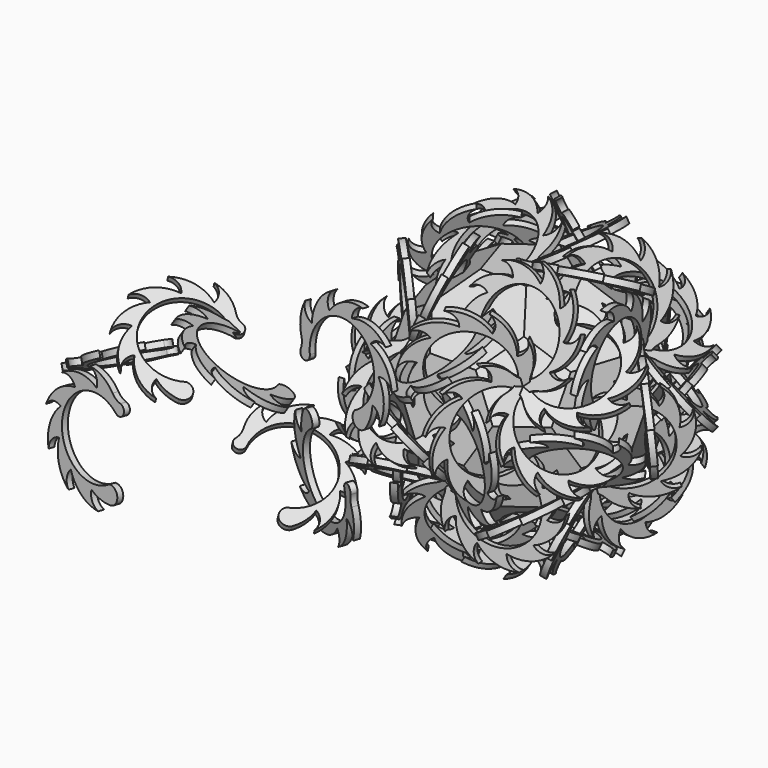
from build123d import *

# Parameters (mm, degrees)
F2_DEPTH  = 1
F3_DEPTH  = 1
F4_ANGLE  = -37.377368
F6_COUNT  = 5
F6_ANGLE  = 288
F9_DEPTH  = 2
F10_R     = 5.4550197089
F12_ANGLE = 65
F13_COUNT = 5
F13_ANGLE = 288
F15_COUNT = 3
F15_ANGLE = 240
F16_COUNT = 5
F16_ANGLE = 288
F17_COUNT = 2
F17_ANGLE = 120
F18_COUNT = 3
F18_ANGLE = 240
F22_COUNT = 3
F22_ANGLE = 144
F26_COUNT = 3
F26_ANGLE = 144
F29_COUNT = 2
F29_ANGLE = 120
F32_COUNT = 3
F32_ANGLE = 144
F36_COUNT = 3
F36_ANGLE = 240
F40_COUNT = 3
F40_ANGLE = 144
F44_COUNT = 3
F44_ANGLE = 144
F48_COUNT = 2
F48_ANGLE = 120
F52_COUNT = 2
F52_ANGLE = 120
F56_COUNT = 2
F56_ANGLE = 120
F60_COUNT = 2
F60_ANGLE = 120


with BuildPart() as f2:
    # F0 (on Top) → F2 (new body)
    with BuildSketch(Plane.XY):
        Polygon((0, -10.3228644035), (7.5, -10.3228644035), (12.1352549156, 3.9429833409), (0, 12.7597621253), align=None)
        Polygon((-7.5, -10.3228644035), (0, -10.3228644035), (0, 12.7597621253), (-12.1352549156, 3.9429833409), align=None)
    extrude(amount=-F2_DEPTH)


with BuildPart() as f3:
    # F1 (on Top) → F3 (new body)
    with BuildSketch(Plane.XY):
        Polygon((32.2091731064, -18.3513614234), (36.844428022, -4.085513679), (26.8074689266, 7.0616587032), (12.1352549156, 3.9429833409), (7.5, -10.3228644035), (17.5369590954, -21.4700367857), align=None)
    extrude(amount=-F3_DEPTH)


with BuildPart() as f3_1:
    # F4: moved
    add(f3.part.rotate(Axis((9.8176274578, -3.1899405313, 0), (-0.3090169944, -0.9510565163, 0)), F4_ANGLE))


with BuildPart() as f6_1:
    # F6: instance of F3
    add(f3_1.part.rotate(Axis((0, 0, 3.8664315362), (0, 0, 1)), 1 * F6_ANGLE / (F6_COUNT - 1)))


with BuildPart() as f6_2:
    # F6: instance of F3
    add(f3_1.part.rotate(Axis((0, 0, 3.8664315362), (0, 0, 1)), 2 * F6_ANGLE / (F6_COUNT - 1)))


with BuildPart() as f6_3:
    # F6: instance of F3
    add(f3_1.part.rotate(Axis((0, 0, 3.8664315362), (0, 0, 1)), 3 * F6_ANGLE / (F6_COUNT - 1)))


with BuildPart() as f6_4:
    # F6: instance of F3
    add(f3_1.part.rotate(Axis((0, 0, 3.8664315362), (0, 0, 1)), 4 * F6_ANGLE / (F6_COUNT - 1)))


with BuildPart() as f9:
    # F8 (on Right) → F9 (new body)
    with BuildSketch(Plane.YZ):
        with BuildLine():
            ThreePointArc((-20.0381562793, -7.4218225341), (-18.0432138806, 14.7456768661), (-1.371596125, 0))
            ThreePointArc((-1.371596125, 0), (1.2710572909, -2.1110060804), (1.0658705895, 1.265065922))
            ThreePointArc((1.0658705895, 1.265065922), (3.462744203, 7.3677169674), (2.5001799222, 13.8531485572))
            ThreePointArc((2.5001799222, 13.8531485572), (1.8396441745, 10.7438611605), (-0.8004298525, 8.9735547684))
            ThreePointArc((-0.8004298525, 8.9735547684), (-2.1304901639, 15.9377846017), (-6.983453041, 21.1067602176))
            ThreePointArc((-6.983453041, 21.1067602176), (-5.7243130519, 18.2607184854), (-6.7542303289, 15.3239417734))
            ThreePointArc((-6.7542303289, 15.3239417734), (-11.923743314, 20.1763322255), (-18.8881203911, 21.5056213332))
            ThreePointArc((-18.8881203911, 21.5056213332), (-16.196593384, 19.9432291213), (-15.3036199233, 16.9619566661))
            ThreePointArc((-15.3036199233, 16.9619566661), (-22.3380073271, 17.8490595111), (-28.7536432712, 14.8309188523))
            ThreePointArc((-28.7536432712, 14.8309188523), (-25.6578010812, 15.1489568819), (-23.1830223937, 13.2619334316))
            ThreePointArc((-23.1830223937, 13.2619334316), (-29.3953873179, 9.8449055341), (-32.8117272579, 3.6321622578))
            ThreePointArc((-32.8117272579, 3.6321622578), (-30.4940763777, 5.7091508113), (-27.3827738075, 5.6371551864))
            ThreePointArc((-27.3827738075, 5.6371551864), (-30.4002040016, -0.7788149372), (-29.5123221974, -7.813104063))
            ThreePointArc((-29.5123221974, -7.813104063), (-28.8581264893, -4.7705040188), (-26.2987118688, -2.9999719366))
            ThreePointArc((-26.2987118688, -2.9999719366), (-26.0274642787, -7.0575500385), (-24.4889350399, -10.821914937))
            ThreePointArc((-24.4889350399, -10.821914937), (-20.5634994581, -11.3472581158), (-20.0381562793, -7.4218225341))
        make_face()
    extrude(amount=-F9_DEPTH)

    # F10
    f10_edges = [f9.edges().sort_by_distance(p)[0] for p in [
        (-1, 1.065871, 1.265066),
    ]]
    fillet(f10_edges, radius=F10_R)


with BuildPart() as f9_1:
    # F12: moved
    add(f9.part.rotate(Axis((0, -10.3228644132, -3.9429833282), (0, -0.9341723595, -0.3568220885)), F12_ANGLE))


with BuildPart() as f13_1:
    # F13: instance of F9
    add(f9_1.part.rotate(Axis((0, 0, 14.2103461549), (0, 0, 1)), 1 * F13_ANGLE / (F13_COUNT - 1)))


with BuildPart() as f13_2:
    # F13: instance of F9
    add(f9_1.part.rotate(Axis((0, 0, 14.2103461549), (0, 0, 1)), 2 * F13_ANGLE / (F13_COUNT - 1)))


with BuildPart() as f13_3:
    # F13: instance of F9
    add(f9_1.part.rotate(Axis((0, 0, 14.2103461549), (0, 0, 1)), 3 * F13_ANGLE / (F13_COUNT - 1)))


with BuildPart() as f13_4:
    # F13: instance of F9
    add(f9_1.part.rotate(Axis((0, 0, 14.2103461549), (0, 0, 1)), 4 * F13_ANGLE / (F13_COUNT - 1)))


with BuildPart() as f15_1:
    # F15: instance of F9
    add(f9_1.part.rotate(Axis((0, -25.3455492518, -1.7338218178), (0, -0.6070619963, 0.7946544738)), 1 * F15_ANGLE / (F15_COUNT - 1)))


with BuildPart() as f15_2:
    # F15: instance of F9
    add(f9_1.part.rotate(Axis((0, -25.3455492518, -1.7338218178), (0, -0.6070619963, 0.7946544738)), 2 * F15_ANGLE / (F15_COUNT - 1)))


with BuildPart() as f16_1:
    # F16: instance of F15_2
    add(f15_2.part.rotate(Axis((0, 0, 14.2103461549), (0, 0, 1)), 1 * F16_ANGLE / (F16_COUNT - 1)))


with BuildPart() as f16_2:
    # F16: instance of F15_2
    add(f15_2.part.rotate(Axis((0, 0, 14.2103461549), (0, 0, 1)), 2 * F16_ANGLE / (F16_COUNT - 1)))


with BuildPart() as f16_3:
    # F16: instance of F15_2
    add(f15_2.part.rotate(Axis((0, 0, 14.2103461549), (0, 0, 1)), 3 * F16_ANGLE / (F16_COUNT - 1)))


with BuildPart() as f16_4:
    # F16: instance of F15_2
    add(f15_2.part.rotate(Axis((0, 0, 14.2103461549), (0, 0, 1)), 4 * F16_ANGLE / (F16_COUNT - 1)))


with BuildPart() as f16_5:
    # F16: instance of F15_1
    add(f15_1.part.rotate(Axis((0, 0, 14.2103461549), (0, 0, 1)), 1 * F16_ANGLE / (F16_COUNT - 1)))


with BuildPart() as f16_6:
    # F16: instance of F15_1
    add(f15_1.part.rotate(Axis((0, 0, 14.2103461549), (0, 0, 1)), 2 * F16_ANGLE / (F16_COUNT - 1)))


with BuildPart() as f16_7:
    # F16: instance of F15_1
    add(f15_1.part.rotate(Axis((0, 0, 14.2103461549), (0, 0, 1)), 3 * F16_ANGLE / (F16_COUNT - 1)))


with BuildPart() as f16_8:
    # F16: instance of F15_1
    add(f15_1.part.rotate(Axis((0, 0, 14.2103461549), (0, 0, 1)), 4 * F16_ANGLE / (F16_COUNT - 1)))


with BuildPart() as f17_1:
    # F17: instance of F3
    add(f3_1.part.rotate(Axis((0, -25.3455492518, -1.7338218178), (0, 0.6070619963, -0.7946544738)), 1 * F17_ANGLE / (F17_COUNT - 1)))


with BuildPart() as f17_2:
    # F17: instance of F16_5
    add(f16_5.part.rotate(Axis((0, -25.3455492518, -1.7338218178), (0, 0.6070619963, -0.7946544738)), 1 * F17_ANGLE / (F17_COUNT - 1)))


with BuildPart() as f17_3:
    # F17: instance of F13_1
    add(f13_1.part.rotate(Axis((0, -25.3455492518, -1.7338218178), (0, 0.6070619963, -0.7946544738)), 1 * F17_ANGLE / (F17_COUNT - 1)))


with BuildPart() as f17_4:
    # F17: instance of F16_1
    add(f16_1.part.rotate(Axis((0, -25.3455492518, -1.7338218178), (0, 0.6070619963, -0.7946544738)), 1 * F17_ANGLE / (F17_COUNT - 1)))


with BuildPart() as f18_1:
    # F18: instance of F2
    add(f2.part.rotate(Axis((0, -25.3455492518, -1.7338218178), (0, -0.6070619963, 0.7946544738)), 1 * F18_ANGLE / (F18_COUNT - 1)))


with BuildPart() as f18_2:
    # F18: instance of F2
    add(f2.part.rotate(Axis((0, -25.3455492518, -1.7338218178), (0, -0.6070619963, 0.7946544738)), 2 * F18_ANGLE / (F18_COUNT - 1)))


with BuildPart() as f18_3:
    # F18: instance of F13_2
    add(f13_2.part.rotate(Axis((0, -25.3455492518, -1.7338218178), (0, -0.6070619963, 0.7946544738)), 1 * F18_ANGLE / (F18_COUNT - 1)))


with BuildPart() as f18_4:
    # F18: instance of F13_2
    add(f13_2.part.rotate(Axis((0, -25.3455492518, -1.7338218178), (0, -0.6070619963, 0.7946544738)), 2 * F18_ANGLE / (F18_COUNT - 1)))


with BuildPart() as f18_5:
    # F18: instance of F13_3
    add(f13_3.part.rotate(Axis((0, -25.3455492518, -1.7338218178), (0, -0.6070619963, 0.7946544738)), 1 * F18_ANGLE / (F18_COUNT - 1)))


with BuildPart() as f18_6:
    # F18: instance of F13_3
    add(f13_3.part.rotate(Axis((0, -25.3455492518, -1.7338218178), (0, -0.6070619963, 0.7946544738)), 2 * F18_ANGLE / (F18_COUNT - 1)))


with BuildPart() as f22_1:
    # F22: instance of F17_1
    add(f17_1.part.rotate(Axis((-18.9711930891, -26.1116072266, -18.7737157723), (0.5257311104, 0.7236067968, -0.4472135991)), 1 * F22_ANGLE / (F22_COUNT - 1)))


with BuildPart() as f22_2:
    # F22: instance of F17_1
    add(f17_1.part.rotate(Axis((-18.9711930891, -26.1116072266, -18.7737157723), (0.5257311104, 0.7236067968, -0.4472135991)), 2 * F22_ANGLE / (F22_COUNT - 1)))


with BuildPart() as f22_3:
    # F22: instance of F17_3
    add(f17_3.part.rotate(Axis((-18.9711930891, -26.1116072266, -18.7737157723), (0.5257311104, 0.7236067968, -0.4472135991)), 1 * F22_ANGLE / (F22_COUNT - 1)))


with BuildPart() as f22_4:
    # F22: instance of F17_3
    add(f17_3.part.rotate(Axis((-18.9711930891, -26.1116072266, -18.7737157723), (0.5257311104, 0.7236067968, -0.4472135991)), 2 * F22_ANGLE / (F22_COUNT - 1)))


with BuildPart() as f22_5:
    # F22: instance of F17_4
    add(f17_4.part.rotate(Axis((-18.9711930891, -26.1116072266, -18.7737157723), (0.5257311104, 0.7236067968, -0.4472135991)), 1 * F22_ANGLE / (F22_COUNT - 1)))


with BuildPart() as f22_6:
    # F22: instance of F17_4
    add(f17_4.part.rotate(Axis((-18.9711930891, -26.1116072266, -18.7737157723), (0.5257311104, 0.7236067968, -0.4472135991)), 2 * F22_ANGLE / (F22_COUNT - 1)))


with BuildPart() as f22_7:
    # F22: instance of F17_2
    add(f17_2.part.rotate(Axis((-18.9711930891, -26.1116072266, -18.7737157723), (0.5257311104, 0.7236067968, -0.4472135991)), 1 * F22_ANGLE / (F22_COUNT - 1)))


with BuildPart() as f22_8:
    # F22: instance of F17_2
    add(f17_2.part.rotate(Axis((-18.9711930891, -26.1116072266, -18.7737157723), (0.5257311104, 0.7236067968, -0.4472135991)), 2 * F22_ANGLE / (F22_COUNT - 1)))


with BuildPart() as f26_1:
    # F26: instance of F3
    add(f3_1.part.rotate(Axis((20.2758098134, -27.9072581024, -17.6639424888), (-0.5257311104, 0.7236067968, -0.4472135991)), 1 * F26_ANGLE / (F26_COUNT - 1)))


with BuildPart() as f26_2:
    # F26: instance of F3
    add(f3_1.part.rotate(Axis((20.2758098134, -27.9072581024, -17.6639424888), (-0.5257311104, 0.7236067968, -0.4472135991)), 2 * F26_ANGLE / (F26_COUNT - 1)))


with BuildPart() as f26_3:
    # F26: instance of F16_1
    add(f16_1.part.rotate(Axis((20.2758098134, -27.9072581024, -17.6639424888), (-0.5257311104, 0.7236067968, -0.4472135991)), 1 * F26_ANGLE / (F26_COUNT - 1)))


with BuildPart() as f26_4:
    # F26: instance of F16_1
    add(f16_1.part.rotate(Axis((20.2758098134, -27.9072581024, -17.6639424888), (-0.5257311104, 0.7236067968, -0.4472135991)), 2 * F26_ANGLE / (F26_COUNT - 1)))


with BuildPart() as f26_5:
    # F26: instance of F13_1
    add(f13_1.part.rotate(Axis((20.2758098134, -27.9072581024, -17.6639424888), (-0.5257311104, 0.7236067968, -0.4472135991)), 1 * F26_ANGLE / (F26_COUNT - 1)))


with BuildPart() as f26_6:
    # F26: instance of F13_1
    add(f13_1.part.rotate(Axis((20.2758098134, -27.9072581024, -17.6639424888), (-0.5257311104, 0.7236067968, -0.4472135991)), 2 * F26_ANGLE / (F26_COUNT - 1)))


with BuildPart() as f26_7:
    # F26: instance of F16_5
    add(f16_5.part.rotate(Axis((20.2758098134, -27.9072581024, -17.6639424888), (-0.5257311104, 0.7236067968, -0.4472135991)), 1 * F26_ANGLE / (F26_COUNT - 1)))


with BuildPart() as f26_8:
    # F26: instance of F16_5
    add(f16_5.part.rotate(Axis((20.2758098134, -27.9072581024, -17.6639424888), (-0.5257311104, 0.7236067968, -0.4472135991)), 2 * F26_ANGLE / (F26_COUNT - 1)))


with BuildPart() as f29_1:
    # F29: instance of F18_2
    add(f18_2.part.rotate(Axis((0, -40.5030693029, -27.1761785704), (0, 0.9822469455, -0.1875924789)), 1 * F29_ANGLE / (F29_COUNT - 1)))


with BuildPart() as f32_1:
    # F32: instance of F26_2
    add(f26_2.part.rotate(Axis((0, -41.1465715097, -55.4848620892), (0, 0.8944271941, 0.4472135893)), 1 * F32_ANGLE / (F32_COUNT - 1)))


with BuildPart() as f32_2:
    # F32: instance of F26_2
    add(f26_2.part.rotate(Axis((0, -41.1465715097, -55.4848620892), (0, 0.8944271941, 0.4472135893)), 2 * F32_ANGLE / (F32_COUNT - 1)))


with BuildPart() as f32_3:
    # F32: instance of F26_4
    add(f26_4.part.rotate(Axis((0, -41.1465715097, -55.4848620892), (0, 0.8944271941, 0.4472135893)), 1 * F32_ANGLE / (F32_COUNT - 1)))


with BuildPart() as f32_4:
    # F32: instance of F26_4
    add(f26_4.part.rotate(Axis((0, -41.1465715097, -55.4848620892), (0, 0.8944271941, 0.4472135893)), 2 * F32_ANGLE / (F32_COUNT - 1)))


with BuildPart() as f32_5:
    # F32: instance of F26_6
    add(f26_6.part.rotate(Axis((0, -41.1465715097, -55.4848620892), (0, 0.8944271941, 0.4472135893)), 1 * F32_ANGLE / (F32_COUNT - 1)))


with BuildPart() as f32_6:
    # F32: instance of F26_6
    add(f26_6.part.rotate(Axis((0, -41.1465715097, -55.4848620892), (0, 0.8944271941, 0.4472135893)), 2 * F32_ANGLE / (F32_COUNT - 1)))


with BuildPart() as f32_7:
    # F32: instance of F18_4
    add(f18_4.part.rotate(Axis((0, -41.1465715097, -55.4848620892), (0, 0.8944271941, 0.4472135893)), 1 * F32_ANGLE / (F32_COUNT - 1)))


with BuildPart() as f32_8:
    # F32: instance of F18_4
    add(f18_4.part.rotate(Axis((0, -41.1465715097, -55.4848620892), (0, 0.8944271941, 0.4472135893)), 2 * F32_ANGLE / (F32_COUNT - 1)))


with BuildPart() as f36_1:
    # F36: instance of F2
    add(f2.part.rotate(Axis((-17.4030966331, 23.953307566, 3.8456892929), (0.3568220886, -0.4911234716, -0.7946544738)), 1 * F36_ANGLE / (F36_COUNT - 1)))


with BuildPart() as f36_2:
    # F36: instance of F2
    add(f2.part.rotate(Axis((-17.4030966331, 23.953307566, 3.8456892929), (0.3568220886, -0.4911234716, -0.7946544738)), 2 * F36_ANGLE / (F36_COUNT - 1)))


with BuildPart() as f40_1:
    # F40: instance of F22_2
    add(f22_2.part.rotate(Axis((-43.9943598437, 14.2946340797, -11.7823727251), (0.8506508064, -0.2763932025, -0.4472135991)), 1 * F40_ANGLE / (F40_COUNT - 1)))


with BuildPart() as f40_2:
    # F40: instance of F22_2
    add(f22_2.part.rotate(Axis((-43.9943598437, 14.2946340797, -11.7823727251), (0.8506508064, -0.2763932025, -0.4472135991)), 2 * F40_ANGLE / (F40_COUNT - 1)))


with BuildPart() as f40_3:
    # F40: instance of F22_6
    add(f22_6.part.rotate(Axis((-43.9943598437, 14.2946340797, -11.7823727251), (0.8506508064, -0.2763932025, -0.4472135991)), 1 * F40_ANGLE / (F40_COUNT - 1)))


with BuildPart() as f40_4:
    # F40: instance of F22_6
    add(f22_6.part.rotate(Axis((-43.9943598437, 14.2946340797, -11.7823727251), (0.8506508064, -0.2763932025, -0.4472135991)), 2 * F40_ANGLE / (F40_COUNT - 1)))


with BuildPart() as f40_5:
    # F40: instance of F22_4
    add(f22_4.part.rotate(Axis((-43.9943598437, 14.2946340797, -11.7823727251), (0.8506508064, -0.2763932025, -0.4472135991)), 1 * F40_ANGLE / (F40_COUNT - 1)))


with BuildPart() as f40_6:
    # F40: instance of F22_4
    add(f22_4.part.rotate(Axis((-43.9943598437, 14.2946340797, -11.7823727251), (0.8506508064, -0.2763932025, -0.4472135991)), 2 * F40_ANGLE / (F40_COUNT - 1)))


with BuildPart() as f40_7:
    # F40: instance of F18_3
    add(f18_3.part.rotate(Axis((-43.9943598437, 14.2946340797, -11.7823727251), (0.8506508064, -0.2763932025, -0.4472135991)), 1 * F40_ANGLE / (F40_COUNT - 1)))


with BuildPart() as f40_8:
    # F40: instance of F18_3
    add(f18_3.part.rotate(Axis((-43.9943598437, 14.2946340797, -11.7823727251), (0.8506508064, -0.2763932025, -0.4472135991)), 2 * F40_ANGLE / (F40_COUNT - 1)))


with BuildPart() as f44_1:
    # F44: instance of F40_2
    add(f40_2.part.rotate(Axis((1.534e-07, 54.8190866503, -7.5020330917), (-6.9e-09, -0.8944271892, -0.4472135991)), 1 * F44_ANGLE / (F44_COUNT - 1)))


with BuildPart() as f44_2:
    # F44: instance of F40_2
    add(f40_2.part.rotate(Axis((1.534e-07, 54.8190866503, -7.5020330917), (-6.9e-09, -0.8944271892, -0.4472135991)), 2 * F44_ANGLE / (F44_COUNT - 1)))


with BuildPart() as f44_3:
    # F44: instance of F40_6
    add(f40_6.part.rotate(Axis((1.534e-07, 54.8190866503, -7.5020330917), (-6.9e-09, -0.8944271892, -0.4472135991)), 1 * F44_ANGLE / (F44_COUNT - 1)))


with BuildPart() as f44_4:
    # F44: instance of F40_6
    add(f40_6.part.rotate(Axis((1.534e-07, 54.8190866503, -7.5020330917), (-6.9e-09, -0.8944271892, -0.4472135991)), 2 * F44_ANGLE / (F44_COUNT - 1)))


with BuildPart() as f44_5:
    # F44: instance of F40_8
    add(f40_8.part.rotate(Axis((1.534e-07, 54.8190866503, -7.5020330917), (-6.9e-09, -0.8944271892, -0.4472135991)), 1 * F44_ANGLE / (F44_COUNT - 1)))


with BuildPart() as f44_6:
    # F44: instance of F40_8
    add(f40_8.part.rotate(Axis((1.534e-07, 54.8190866503, -7.5020330917), (-6.9e-09, -0.8944271892, -0.4472135991)), 2 * F44_ANGLE / (F44_COUNT - 1)))


with BuildPart() as f44_7:
    # F44: instance of F40_4
    add(f40_4.part.rotate(Axis((1.534e-07, 54.8190866503, -7.5020330917), (-6.9e-09, -0.8944271892, -0.4472135991)), 1 * F44_ANGLE / (F44_COUNT - 1)))


with BuildPart() as f44_8:
    # F44: instance of F40_4
    add(f40_4.part.rotate(Axis((1.534e-07, 54.8190866503, -7.5020330917), (-6.9e-09, -0.8944271892, -0.4472135991)), 2 * F44_ANGLE / (F44_COUNT - 1)))


with BuildPart() as f48_1:
    # F48: instance of F22_2
    add(f22_2.part.rotate(Axis((-45.320051719, 14.7253777202, -44.0123603845), (0.9341723533, -0.3035310175, 0.1875924726)), 1 * F48_ANGLE / (F48_COUNT - 1)))


with BuildPart() as f48_2:
    # F48: instance of F22_4
    add(f22_4.part.rotate(Axis((-45.320051719, 14.7253777202, -44.0123603845), (0.9341723533, -0.3035310175, 0.1875924726)), 1 * F48_ANGLE / (F48_COUNT - 1)))


with BuildPart() as f48_3:
    # F48: instance of F22_6
    add(f22_6.part.rotate(Axis((-45.320051719, 14.7253777202, -44.0123603845), (0.9341723533, -0.3035310175, 0.1875924726)), 1 * F48_ANGLE / (F48_COUNT - 1)))


with BuildPart() as f48_4:
    # F48: instance of F18_3
    add(f18_3.part.rotate(Axis((-45.320051719, 14.7253777202, -44.0123603845), (0.9341723533, -0.3035310175, 0.1875924726)), 1 * F48_ANGLE / (F48_COUNT - 1)))


with BuildPart() as f52_1:
    # F52: instance of F16_5
    add(f16_5.part.rotate(Axis((51.1630279448, -16.6238756598, -24.6374564773), (-0.9341723577, 0.3035310035, -0.1875924733)), 1 * F52_ANGLE / (F52_COUNT - 1)))


with BuildPart() as f52_2:
    # F52: instance of F13_1
    add(f13_1.part.rotate(Axis((51.1630279448, -16.6238756598, -24.6374564773), (-0.9341723577, 0.3035310035, -0.1875924733)), 1 * F52_ANGLE / (F52_COUNT - 1)))


with BuildPart() as f52_3:
    # F52: instance of F16_1
    add(f16_1.part.rotate(Axis((51.1630279448, -16.6238756598, -24.6374564773), (-0.9341723577, 0.3035310035, -0.1875924733)), 1 * F52_ANGLE / (F52_COUNT - 1)))


with BuildPart() as f52_4:
    # F52: instance of F3
    add(f3_1.part.rotate(Axis((51.1630279448, -16.6238756598, -24.6374564773), (-0.9341723577, 0.3035310035, -0.1875924733)), 1 * F52_ANGLE / (F52_COUNT - 1)))


with BuildPart() as f56_1:
    # F56: instance of F26_2
    add(f26_2.part.rotate(Axis((20.2389789509, -27.8565650407, -79.9844450272), (-0.3568220897, 0.4911234788, 0.7946544689)), 1 * F56_ANGLE / (F56_COUNT - 1)))


with BuildPart() as f56_2:
    # F56: instance of F26_4
    add(f26_4.part.rotate(Axis((20.2389789509, -27.8565650407, -79.9844450272), (-0.3568220897, 0.4911234788, 0.7946544689)), 1 * F56_ANGLE / (F56_COUNT - 1)))


with BuildPart() as f56_3:
    # F56: instance of F26_6
    add(f26_6.part.rotate(Axis((20.2389789509, -27.8565650407, -79.9844450272), (-0.3568220897, 0.4911234788, 0.7946544689)), 1 * F56_ANGLE / (F56_COUNT - 1)))


with BuildPart() as f56_4:
    # F56: instance of F18_4
    add(f18_4.part.rotate(Axis((20.2389789509, -27.8565650407, -79.9844450272), (-0.3568220897, 0.4911234788, 0.7946544689)), 1 * F56_ANGLE / (F56_COUNT - 1)))


with BuildPart() as f60_1:
    # F60: instance of F52_4
    add(f52_4.part.rotate(Axis((24.2012826257, 7.8634731584, -68.221784607), (-0.5773502692, -0.1875924683, 0.7946544737)), 1 * F60_ANGLE / (F60_COUNT - 1)))


with BuildPart() as f60_2:
    # F60: instance of F52_3
    add(f52_3.part.rotate(Axis((24.2012826257, 7.8634731584, -68.221784607), (-0.5773502692, -0.1875924683, 0.7946544737)), 1 * F60_ANGLE / (F60_COUNT - 1)))


with BuildPart() as f60_3:
    # F60: instance of F52_1
    add(f52_1.part.rotate(Axis((24.2012826257, 7.8634731584, -68.221784607), (-0.5773502692, -0.1875924683, 0.7946544737)), 1 * F60_ANGLE / (F60_COUNT - 1)))


with BuildPart() as f60_4:
    # F60: instance of F52_2
    add(f52_2.part.rotate(Axis((24.2012826257, 7.8634731584, -68.221784607), (-0.5773502692, -0.1875924683, 0.7946544737)), 1 * F60_ANGLE / (F60_COUNT - 1)))


with BuildPart() as f9_2:
    # F65: moved
    add(f9_1.part.moved(Location((-36, -74.6, 0))))


with BuildPart() as f13_1_1:
    # F65: moved
    add(f13_1.part.moved(Location((-36, -74.6, 0))))


with BuildPart() as f16_8_1:
    # F65: moved
    add(f16_8.part.moved(Location((-36, -74.6, 0))))


with BuildPart() as f44_4_1:
    # F65: moved
    add(f44_4.part.moved(Location((-36, -74.6, 0))))


with BuildPart() as f60_3_1:
    # F65: moved
    add(f60_3.part.moved(Location((-36, -74.6, 0))))


with BuildPart() as f18_5_1:
    # F65: moved
    add(f18_5.part.moved(Location((-36, -74.6, 0))))


with BuildPart() as f44_5_1:
    # F65: moved
    add(f44_5.part.moved(Location((-36, -74.6, 0))))


solid = Compound([f2.part, f3_1.part, f6_1.part, f6_2.part, f6_3.part, f6_4.part, f13_2.part, f13_3.part, f13_4.part, f15_1.part, f15_2.part, f16_1.part, f16_2.part, f16_3.part, f16_4.part, f16_5.part, f16_6.part, f16_7.part, f17_1.part, f17_2.part, f17_3.part, f17_4.part, f18_1.part, f18_2.part, f18_3.part, f18_4.part, f18_6.part, f22_1.part, f22_2.part, f22_3.part, f22_4.part, f22_5.part, f22_6.part, f26_1.part, f26_2.part, f26_3.part, f26_4.part, f26_5.part, f26_6.part, f29_1.part, f32_1.part, f32_2.part, f32_3.part, f32_4.part, f32_5.part, f32_6.part, f32_7.part, f32_8.part, f36_1.part, f36_2.part, f40_1.part, f40_2.part, f40_3.part, f40_4.part, f40_5.part, f40_6.part, f40_7.part, f40_8.part, f44_1.part, f44_2.part, f44_3.part, f44_6.part, f44_7.part, f44_8.part, f48_1.part, f48_2.part, f48_3.part, f48_4.part, f52_1.part, f52_2.part, f52_3.part, f52_4.part, f56_1.part, f56_2.part, f56_3.part, f56_4.part, f60_1.part, f60_2.part, f60_4.part, f9_2.part, f13_1_1.part, f16_8_1.part, f44_4_1.part, f60_3_1.part, f18_5_1.part, f44_5_1.part])
